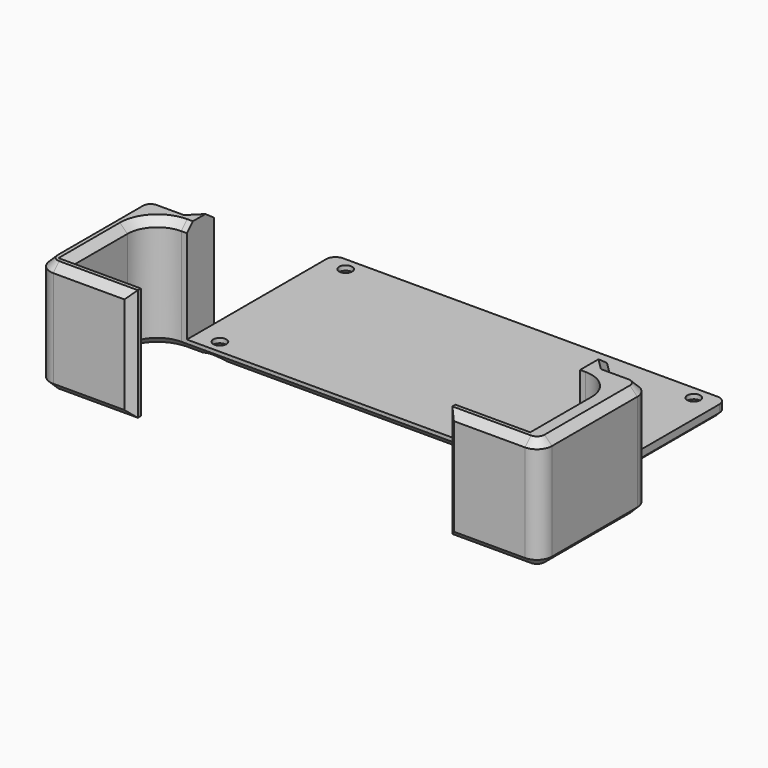
from build123d import *

# Parameters (mm, degrees)
F1_DEPTH       = 30
F3_DEPTH       = 27
F4_SIZE        = 2
F5_SIZE        = 2
F7_D           = 3.5
F7_CSINK_D     = 7
F7_CSINK_ANGLE = 90
F8_T1_DEPTH    = 108
F8_T6_DEPTH    = 25.6433659759
F8_T12_DEPTH   = 25.6433659759
F8_T17_DEPTH   = 25.6433659759
F8_T22_DEPTH   = 25.6433659759
F8_T26_ANGLE   = 90
F8_T28_ANGLE   = 90
F9_T1_DEPTH    = 100
F9_T6_DEPTH    = 40.0716830997
F9_T11_DEPTH   = 13.6286473502
F9_T17_DEPTH   = 13.6286473502
F9_T21_ANGLE   = 90
F9_T23_ANGLE   = 90
F9_T27_DEPTH   = 40.0716830997
F9_T33_DEPTH   = 13.6286473502
F9_T37_DEPTH   = 40.0716830997
F9_T44_DEPTH   = 40.0716830997
F9_T48_DEPTH   = 13.6286473502


# Not quite as in the source:
# - a fillet or chamfer that OpenCascade refuses, or shapes differently, is made with other operations: its cross-section is extruded or revolved along the edge and cut away or added


with BuildPart() as f1:
    # F0 (on Top) → F1 (new body)
    with BuildSketch(Plane.XY):
        with BuildLine():
            Line((-1.5, 0), (0, 0))
            Line((0, 0), (105, 0))
            Line((105, 0), (106.5, 0))
            ThreePointArc((106.5, 0), (112.1568542495, -2.3431457505), (114.5, -8))
            Line((114.5, -8), (114.5, -26.5))
            Line((114.5, -26.5), (94.5, -26.5))
            Line((94.5, -26.5), (94.5, -31.4999998882))
            Line((94.5, -31.4999998882), (115.4999998882, -31.4999998882))
            ThreePointArc((115.4999998882, -31.4999998882), (118.328427013, -30.328427013), (119.4999998882, -27.4999998882))
            Line((119.4999998882, -27.4999998882), (119.4999998882, 0.9999998882))
            ThreePointArc((119.4999998882, 0.9999998882), (118.328427013, 3.828427013), (115.4999998882, 4.9999998882))
            Line((115.4999998882, 4.9999998882), (109, 4.9999998882))
            Line((109, 4.9999998882), (105, 8.9999998882))
            Line((105, 8.9999998882), (105, 46.5))
            ThreePointArc((105, 46.5), (104.267766953, 48.267766953), (102.5, 49))
            Line((102.5, 49), (2.5, 49))
            ThreePointArc((2.5, 49), (0.732233047, 48.267766953), (0, 46.5))
            Line((0, 46.5), (0, 8.9999998882))
            Line((0, 8.9999998882), (-4, 4.9999998882))
            Line((-4, 4.9999998882), (-10.4999998882, 4.9999998882))
            ThreePointArc((-10.4999998882, 4.9999998882), (-13.328427013, 3.828427013), (-14.4999998882, 0.9999998882))
            Line((-14.4999998882, 0.9999998882), (-14.4999998882, -27.4999998882))
            ThreePointArc((-14.4999998882, -27.4999998882), (-13.328427013, -30.328427013), (-10.4999998882, -31.4999998882))
            Line((-10.4999998882, -31.4999998882), (10.5, -31.4999998882))
            Line((10.5, -31.4999998882), (10.5, -26.5))
            Line((10.5, -26.5), (-9.5, -26.5))
            Line((-9.5, -26.5), (-9.5, -8))
            ThreePointArc((-9.5, -8), (-7.1568542495, -2.3431457505), (-1.5, 0))
        make_face()
    extrude(amount=F1_DEPTH)

    # F2 (on face) → F3 (cut)
    with BuildSketch(Plane.XY.offset(30)):
        with BuildLine():
            Line((0, 0), (105, 0))
            Line((105, 0), (105, 4.9999998882))
            Line((105, 4.9999998882), (105, 8.9999998882))
            Line((105, 8.9999998882), (105, 46.5))
            ThreePointArc((105, 46.5), (104.267766953, 48.267766953), (102.5, 49))
            Line((102.5, 49), (2.5, 49))
            ThreePointArc((2.5, 49), (0.732233047, 48.267766953), (0, 46.5))
            Line((0, 46.5), (0, 8.9999998882))
            Line((0, 8.9999998882), (0, 4.9999998882))
            Line((0, 4.9999998882), (0, 0))
        make_face()
    extrude(amount=-F3_DEPTH, mode=Mode.SUBTRACT)

    # F4
    f4_edges = [f1.edges().sort_by_distance(p)[0] for p in [
        (94.5, -26.5, 15),
        (94.5, -31.5, 15),
        (10.5, -31.5, 15),
        (10.5, -26.5, 15),
    ]]
    chamfer(f4_edges, length=F4_SIZE)

    # F5
    f5_edges = [f1.edges().sort_by_distance(p)[0] for p in [
        (105.5, -26.5, 0),
        (-0.5, -26.5, 0),
        (-1, -31.5, 0),
        (106, -31.5, 0),
        (-7.25, 5, 30),
        (-9.5, -17.25, 30),
        (-0.5, -26.5, 30),
        (105.5, -26.5, 30),
        (106, -31.5, 30),
        (107, 7, 30),
        (-2, 7, 30),
    ]]
    chamfer(f5_edges, length=F5_SIZE)

    # F7 (through all)
    with Locations(Plane(origin=(0, 0, 0), x_dir=(1, 0, 0), z_dir=(0, 0, -1))):
        with Locations((6, -3.5), (6, -45.5), (99, -3.5), (99, -45.5)):
            CounterSinkHole(F7_D / 2, F7_CSINK_D / 2, counter_sink_angle=F7_CSINK_ANGLE)

    # F8: chamfer of 2 on 5 edges, made by hand

    # F8_s2 → F8_t1 (cut)
    with BuildSketch(Plane.YZ.offset(-1.5)):
        Polygon((2, 0), (0, 2), (0, 0), align=None)
    extrude(amount=F8_T1_DEPTH, mode=Mode.SUBTRACT)


with BuildPart() as f8_tool4:
    # F8_s5 → F8_t6 (new body)
    with BuildSketch(Plane.XZ.offset(33.6433659759)):
        Polygon((116.5, 0), (114.5, 2), (114.5, 0), align=None)
    extrude(amount=-F8_T6_DEPTH)

    split(bisect_by=Plane.XZ.offset(26.5), keep=Keep.TOP)

    split(bisect_by=Plane(origin=(0, -14.25, 14.25), x_dir=(1, 0, 0), z_dir=(0, 0.7071067812, -0.7071067812)), keep=Keep.TOP)


with BuildPart() as f1_1:
    add(f1.part)

    # F8_t3: cut F8_tool4
    add(f8_tool4.part, mode=Mode.SUBTRACT)


with BuildPart() as f8_tool10:
    # F8_s11 → F8_t12 (new body)
    with BuildSketch(Plane.XZ.offset(33.6433659759)):
        Polygon((116.5, 0), (114.5, 2), (114.5, 0), align=None)
    extrude(amount=-F8_T12_DEPTH)

    split(bisect_by=Plane.XZ.offset(26.5), keep=Keep.BOTTOM)


with BuildPart() as f1_2:
    add(f1_1.part)

    # F8_t9: cut F8_tool10
    add(f8_tool10.part, mode=Mode.SUBTRACT)


with BuildPart() as f8_tool15:
    # F8_s16 → F8_t17 (new body)
    with BuildSketch(Plane.XZ.offset(8)):
        Polygon((-11.5, 0), (-9.5, 2), (-9.5, 0), align=None)
    extrude(amount=F8_T17_DEPTH)

    split(bisect_by=Plane.XZ.offset(26.5), keep=Keep.BOTTOM)


with BuildPart() as f1_3:
    add(f1_2.part)

    # F8_t14: cut F8_tool15
    add(f8_tool15.part, mode=Mode.SUBTRACT)


with BuildPart() as f8_tool20:
    # F8_s21 → F8_t22 (new body)
    with BuildSketch(Plane.XZ.offset(8)):
        Polygon((-11.5, 0), (-9.5, 2), (-9.5, 0), align=None)
    extrude(amount=F8_T22_DEPTH)

    split(bisect_by=Plane.XZ.offset(26.5), keep=Keep.TOP)

    split(bisect_by=Plane(origin=(0, -14.25, 14.25), x_dir=(1, 0, 0), z_dir=(0, 0.7071067812, -0.7071067812)), keep=Keep.TOP)


with BuildPart() as f1_4:
    add(f1_3.part)

    # F8_t19: cut F8_tool20
    add(f8_tool20.part, mode=Mode.SUBTRACT)

    # F8_s25 → F8_t26 (revolve, cut)
    with BuildSketch(Plane.XZ.offset(8)):
        Polygon((-11.5, 0), (-9.5, 2), (-9.5, 0), align=None)
    revolve(axis=Axis((-1.5, -8, 0), (0, 0, -1)), revolution_arc=F8_T26_ANGLE, mode=Mode.SUBTRACT)

    # F8_s27 → F8_t28 (revolve, cut)
    with BuildSketch(Plane.YZ.offset(106.5)):
        Polygon((2, 0), (0, 2), (0, 0), align=None)
    revolve(axis=Axis((106.5, -8, 0), (0, 0, -1)), revolution_arc=F8_T28_ANGLE, mode=Mode.SUBTRACT)

    # F9: chamfer of 1 on 7 edges, made by hand

    # F9_s2 → F9_t1 (cut)
    with BuildSketch(Plane.YZ.offset(2.5)):
        Polygon((48, 0), (49, 1), (49, 0), align=None)
    extrude(amount=F9_T1_DEPTH, mode=Mode.SUBTRACT)


with BuildPart() as f9_tool4:
    # F9_s5 → F9_t6 (new body)
    with BuildSketch(Plane.XZ.offset(-46.5)):
        Polygon((1, 0), (0, 1), (0, 0), align=None)
    extrude(amount=F9_T6_DEPTH)

    split(bisect_by=Plane(origin=(-4.4999999441, 4.4999999441, 0), x_dir=(0, 0, 1), z_dir=(-0.7071067812, 0.7071067812, 0)), keep=Keep.TOP)


with BuildPart() as f1_5:
    add(f1_4.part)

    # F9_t3: cut F9_tool4
    add(f9_tool4.part, mode=Mode.SUBTRACT)


with BuildPart() as f9_tool9:
    # F9_s10 → F9_t11 (new body)
    with BuildSketch(Plane(origin=(-3.3184545357, -3.3184545357, 0), x_dir=(0, 0, 1), z_dir=(0.7071067812, 0.7071067812, 0))):
        Polygon((0, -5.3639609517), (1, -6.3639609517), (0, -6.3639609517), align=None)
    extrude(amount=F9_T11_DEPTH)

    split(bisect_by=Plane(origin=(0, 1.4999999441, -1.4999999441), x_dir=(1, 0, 0), z_dir=(0, 0.7071067812, -0.7071067812)), keep=Keep.TOP)

    split(bisect_by=Plane.YZ, keep=Keep.BOTTOM)


with BuildPart() as f1_6:
    add(f1_5.part)

    # F9_t8: cut F9_tool9
    add(f9_tool9.part, mode=Mode.SUBTRACT)


with BuildPart() as f9_tool15:
    # F9_s16 → F9_t17 (new body)
    with BuildSketch(Plane(origin=(46.181545576, -46.181545576, 0), x_dir=(0, 0, 1), z_dir=(0.7071067812, -0.7071067812, 0))):
        Polygon((0, -79.6101729762), (1, -80.6101729762), (0, -80.6101729762), align=None)
    extrude(amount=F9_T17_DEPTH)

    split(bisect_by=Plane.YZ.offset(105), keep=Keep.TOP)

    split(bisect_by=Plane(origin=(0, 1.4999999441, -1.4999999441), x_dir=(1, 0, 0), z_dir=(0, 0.7071067812, -0.7071067812)), keep=Keep.TOP)


with BuildPart() as f1_7:
    add(f1_6.part)

    # F9_t14: cut F9_tool15
    add(f9_tool15.part, mode=Mode.SUBTRACT)

    # F9_s20 → F9_t21 (revolve, cut)
    with BuildSketch(Plane.YZ.offset(2.5)):
        Polygon((48, 0), (49, 1), (49, 0), align=None)
    revolve(axis=Axis((2.5, 46.5, 0), (0, 0, 1)), revolution_arc=F9_T21_ANGLE, mode=Mode.SUBTRACT)

    # F9_s22 → F9_t23 (revolve, cut)
    with BuildSketch(Plane.XZ.offset(-46.5)):
        Polygon((104, 0), (105, 1), (105, 0), align=None)
    revolve(axis=Axis((102.5, 46.5, 0), (0, 0, 1)), revolution_arc=F9_T23_ANGLE, mode=Mode.SUBTRACT)


with BuildPart() as f9_tool25:
    # F9_s26 → F9_t27 (new body)
    with BuildSketch(Plane.XZ.offset(-6.4283169003)):
        Polygon((104, 0), (105, 1), (105, 0), align=None)
    extrude(amount=-F9_T27_DEPTH)

    split(bisect_by=Plane(origin=(56.9999999441, 56.9999999441, 0), x_dir=(0, 0, 1), z_dir=(0.7071067812, 0.7071067812, 0)), keep=Keep.TOP)


with BuildPart() as f1_8:
    add(f1_7.part)

    # F9_t24: cut F9_tool25
    add(f9_tool25.part, mode=Mode.SUBTRACT)


with BuildPart() as f9_tool31:
    # F9_s32 → F9_t33 (new body)
    with BuildSketch(Plane(origin=(-3.3184545357, -3.3184545357, 0), x_dir=(0, 0, 1), z_dir=(0.7071067812, 0.7071067812, 0))):
        Polygon((0, -5.3639609517), (1, -6.3639609517), (0, -6.3639609517), align=None)
    extrude(amount=F9_T33_DEPTH)

    split(bisect_by=Plane.YZ, keep=Keep.TOP)


with BuildPart() as f9_tool35:
    # F9_s36 → F9_t37 (new body)
    with BuildSketch(Plane.XZ.offset(-46.5)):
        Polygon((1, 0), (0, 1), (0, 0), align=None)
    extrude(amount=F9_T37_DEPTH)

    split(bisect_by=Plane(origin=(-4.4999999441, 4.4999999441, 0), x_dir=(0, 0, 1), z_dir=(0.7071067812, -0.7071067812, 0)), keep=Keep.TOP)


with BuildPart() as f9_tool31_1:
    add(f9_tool31.part)

    # F9_t39: intersect F9_tool35
    add(f9_tool35.part, mode=Mode.INTERSECT)


with BuildPart() as f1_9:
    add(f1_8.part)

    # F9_t29: cut F9_tool31
    add(f9_tool31_1.part, mode=Mode.SUBTRACT)


with BuildPart() as f9_tool42:
    # F9_s43 → F9_t44 (new body)
    with BuildSketch(Plane.XZ.offset(-6.4283169003)):
        Polygon((104, 0), (105, 1), (105, 0), align=None)
    extrude(amount=-F9_T44_DEPTH)

    split(bisect_by=Plane(origin=(56.9999999441, 56.9999999441, 0), x_dir=(0, 0, 1), z_dir=(-0.7071067812, -0.7071067812, 0)), keep=Keep.TOP)


with BuildPart() as f9_tool46:
    # F9_s47 → F9_t48 (new body)
    with BuildSketch(Plane(origin=(46.181545576, -46.181545576, 0), x_dir=(0, 0, 1), z_dir=(0.7071067812, -0.7071067812, 0))):
        Polygon((0, -79.6101729762), (1, -80.6101729762), (0, -80.6101729762), align=None)
    extrude(amount=F9_T48_DEPTH)

    split(bisect_by=Plane.YZ.offset(105), keep=Keep.BOTTOM)


with BuildPart() as f9_tool42_1:
    add(f9_tool42.part)

    # F9_t50: intersect F9_tool46
    add(f9_tool46.part, mode=Mode.INTERSECT)


with BuildPart() as f1_10:
    add(f1_9.part)

    # F9_t40: cut F9_tool42
    add(f9_tool42_1.part, mode=Mode.SUBTRACT)


solid = f1_10.part
